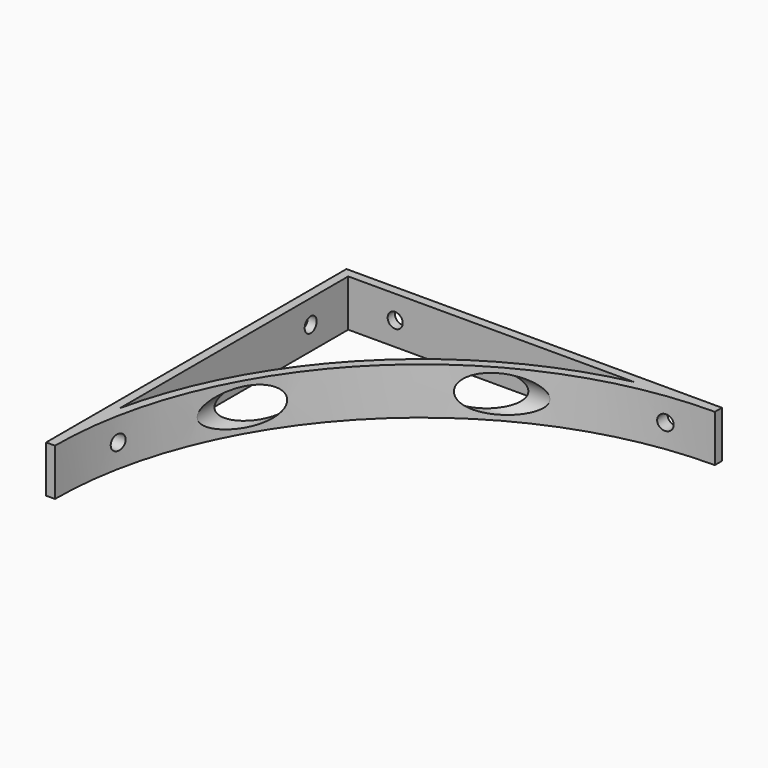
from build123d import *

# Parameters (mm, degrees)
F1_DEPTH = 12.7
F2_R     = 2.032
F3_DEPTH = 101.601
F4_R     = 2.032
F5_DEPTH = 101.601
F6_R     = 4.953
F7_DEPTH = 63.246
F9_START = 18.542
F8_R     = 4.953
F9_DEPTH = 49.53


with BuildPart() as f1:
    # F0 (on Top) → F1 (new body)
    with BuildSketch(Plane.XY):
        with BuildLine():
            Line((101.6, 99.2), (101.6, 101.6))
            Line((101.6, 101.6), (0, 101.6))
            Line((0, 101.6), (0, 0))
            Line((0, 0), (2.4, 0))
            ThreePointArc((2.4, 0), (31.4550073063, 70.1449926937), (101.6, 99.2))
        make_face()
        with BuildLine():
            Line((2.4, 99.2), (79.6473236256, 99.2))
            ThreePointArc((79.6473236256, 99.2), (29.7579510314, 71.8420489686), (2.4, 21.9526763744))
            Line((2.4, 21.9526763744), (2.4, 99.2))
        make_face(mode=Mode.SUBTRACT)
    extrude(amount=F1_DEPTH)

    # F2 (on Right) → F3 (cut, through all)
    with BuildSketch(Plane.YZ):
        with Locations((19.05, 6.35)):
            Circle(F2_R)
        with BuildLine():
            ThreePointArc((88.532, 6.35), (86.5, 8.382), (84.468, 6.35))
            ThreePointArc((84.468, 6.35), (86.5, 4.318), (88.532, 6.35))
        make_face()
    extrude(amount=F3_DEPTH, mode=Mode.SUBTRACT)

    # F4 (on Front) → F5 (cut, through all)
    with BuildSketch(Plane.XZ):
        with Locations((15.1, 6.35)):
            Circle(F4_R)
        with Locations((88.9, 6.35)):
            Circle(F4_R)
    extrude(amount=-F5_DEPTH, mode=Mode.SUBTRACT)

    # F6 (on Front) → F7 (cut)
    with BuildSketch(Plane.XZ):
        with Locations((15.1, 6.35)):
            Circle(F6_R)
    extrude(amount=-F7_DEPTH, mode=Mode.SUBTRACT)

    # F8 (on Right) → F9 (cut)
    with BuildSketch(Plane.YZ.offset(F9_START)):
        with Locations((86.5, 6.35)):
            Circle(F8_R)
    extrude(amount=F9_DEPTH, mode=Mode.SUBTRACT)


solid = f1.part
